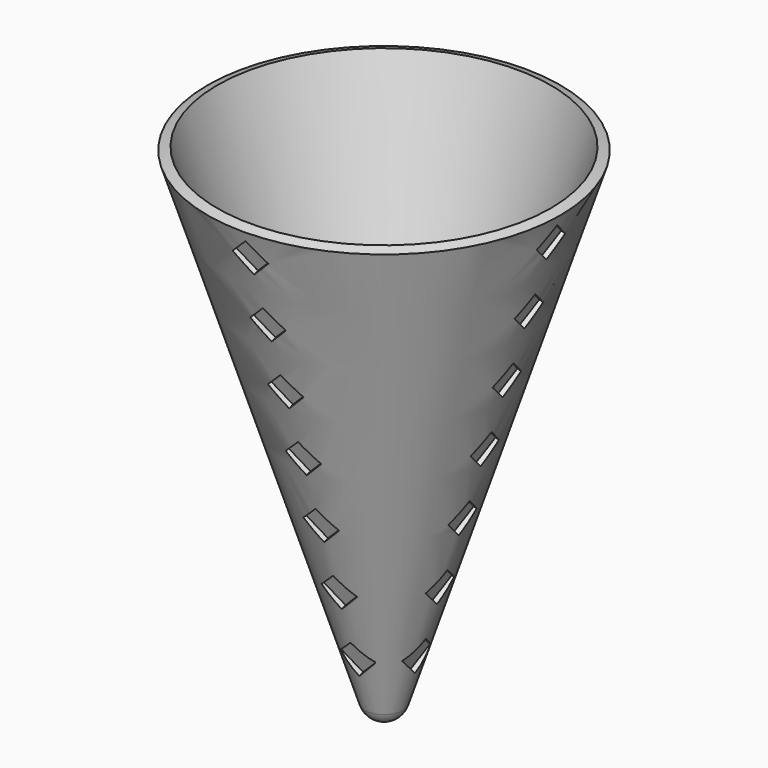
from build123d import *

# Parameters (mm, degrees)
F4_DEPTH        = 1
F4_COPIES_COUNT = 4


# Not quite as in the source:
# - a pattern or mirror of a feature is missing from the dataset's text; its kind, count and spacing are read off the source's solid


with BuildPart() as f1:
    # F0 (on Front) → F1 (revolve)
    with BuildSketch(Plane.XZ):
        with BuildLine():
            Line((0, 11.0187885784), (0, 9.0187885784))
            ThreePointArc((0, 9.0187885784), (2.3541482546, 9.784907629), (3.8065175964, 11.7897955808))
            Line((3.8065175964, 11.7897955808), (35, 108.4042920796))
            Line((35, 108.4042920796), (33.0967412018, 109.0187885784))
            Line((33.0967412018, 109.0187885784), (1.9032587982, 12.4042920796))
            ThreePointArc((1.9032587982, 12.4042920796), (1.1770741273, 11.4018481037), (0, 11.0187885784))
        make_face()
    revolve(axis=Axis((0, 0, 10.0187885784), (0, 0, 1)))

    # F3 (on line) → F4 (cut)
    with BuildSketch(Plane(origin=(0, 0, 0), x_dir=(0, 1, 0), z_dir=(0.9516293991, 0, -0.3072482494))):
        Polygon((0, 111.9144000611), (-3.5355339059, 108.3788661552), (0, 104.8433322492), (3.5355339059, 108.3788661552), align=None)
        Polygon((0, 97.7722644374), (-3.5355339059, 94.2367305314), (0, 90.7011966255), (3.5355339059, 94.2367305314), align=None)
        Polygon((0, 83.6301288136), (-3.5355339059, 80.0945949077), (0, 76.5590610018), (3.5355339059, 80.0945949077), align=None)
        Polygon((0, 69.4879931899), (-3.5355339059, 65.952459284), (0, 62.4169253781), (3.5355339059, 65.952459284), align=None)
        Polygon((0, 55.3458575662), (-3.5355339059, 51.8103236603), (0, 48.2747897543), (3.5355339059, 51.8103236603), align=None)
        Polygon((0, 41.2037219425), (-3.5355339059, 37.6681880365), (0, 34.1326541306), (3.5355339059, 37.6681880365), align=None)
        Polygon((0, 27.0615863187), (-3.5355339059, 23.5260524128), (0, 19.9905185069), (3.5355339059, 23.5260524128), align=None)
    f4 = extrude(amount=-F4_DEPTH, mode=Mode.SUBTRACT)

    # F4_copies: F4 ×4 about axis
    f4_copies_axis = Axis((0, 0, 0), (0, 0, 1))
    for i in range(1, F4_COPIES_COUNT):
        add(f4.rotate(f4_copies_axis, i * 360 / F4_COPIES_COUNT), mode=Mode.SUBTRACT)


solid = f1.part
